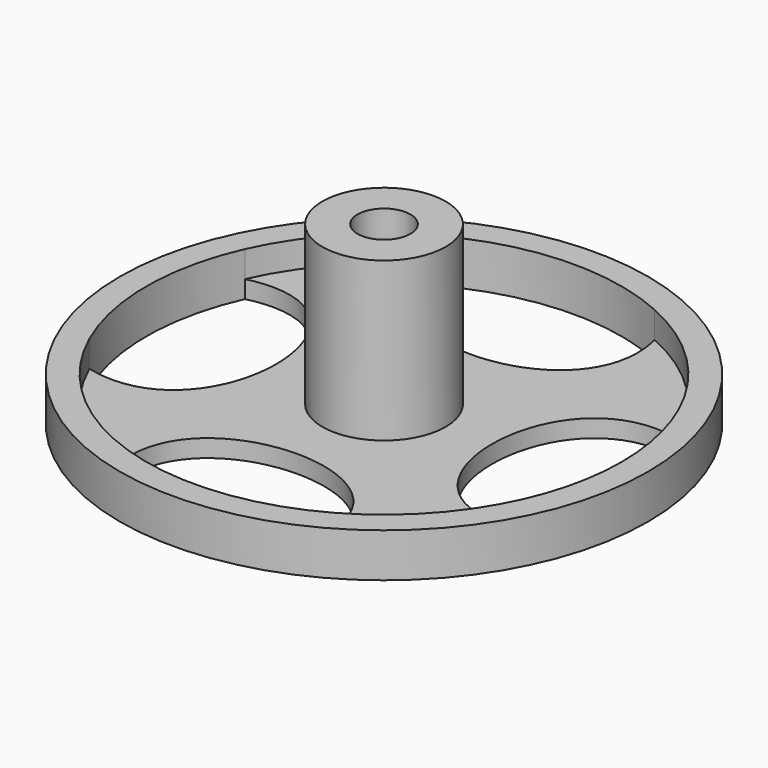
from build123d import *

# Parameters (mm, degrees)
F0_R     = 30
F1_DEPTH = 5
F0_R_2   = 7
F0_R_3   = 3
F2_DEPTH = 2
F3_DEPTH = 15


# Not quite as in the source:
# - a feature names something its author has since deleted; it is built from what else it names


with BuildPart() as f1:
    # F0 (on Top) → F1 (new body)
    with BuildSketch(Plane.XY):
        Circle(F0_R)
        with BuildLine():
            ThreePointArc((24.6394529882, 11.040713584), (26.4032690275, 5.6451204292), (27, 0))
            ThreePointArc((27, 0), (26.4032690275, -5.6451204292), (24.6394529882, -11.040713584))
            ThreePointArc((24.6394529882, -11.040713584), (19.091883092, -19.091883092), (11.040713584, -24.6394529882))
            ThreePointArc((11.040713584, -24.6394529882), (0, -27), (-11.040713584, -24.6394529882))
            ThreePointArc((-11.040713584, -24.6394529882), (-19.091883092, -19.091883092), (-24.6394529882, -11.040713584))
            ThreePointArc((-24.6394529882, -11.040713584), (-27, 0), (-24.6394529882, 11.040713584))
            ThreePointArc((-24.6394529882, 11.040713584), (-19.091883092, 19.091883092), (-11.040713584, 24.6394529882))
            ThreePointArc((-11.040713584, 24.6394529882), (0, 27), (11.040713584, 24.6394529882))
            ThreePointArc((11.040713584, 24.6394529882), (19.091883092, 19.091883092), (24.6394529882, 11.040713584))
        make_face(mode=Mode.SUBTRACT)
    extrude(amount=F1_DEPTH)


with BuildPart() as f1b:
    # F0 (on Top) → F1, piece 2 (new body)
    with BuildSketch(Plane.XY):
        Circle(F0_R_2)
        Circle(F0_R_3, mode=Mode.SUBTRACT)
    extrude(amount=F1_DEPTH)

    # F3 (add): a face of the model
    f3_faces = [f1b.faces().sort_by_distance(p)[0] for p in [
        (-6.8020101013, 0, 5),
    ]]
    extrude(f3_faces, amount=F3_DEPTH)


with BuildPart() as f2:
    # F0 (on Top) → F2 (new body)
    with BuildSketch(Plane.XY):
        with BuildLine():
            add(Edge.make_bspline(
                [(24.6394529882, 11.040713584), (8.1415599535, 15), (8.1415599535, -15), (24.6394529882, -11.040713584)],
                knots=[0, 0, 0, 0, 22.081427168, 22.081427168, 22.081427168, 22.081427168], degree=3))
            ThreePointArc((24.6394529882, 11.040713584), (19.091883092, 19.091883092), (11.040713584, 24.6394529882))
            add(Edge.make_bspline(
                [(-11.040713584, 24.6394529882), (-15, 8.1415599535), (15, 8.1415599535), (11.040713584, 24.6394529882)],
                knots=[0, 0, 0, 0, 22.081427168, 22.081427168, 22.081427168, 22.081427168], degree=3))
            ThreePointArc((-11.040713584, 24.6394529882), (-19.091883092, 19.091883092), (-24.6394529882, 11.040713584))
            add(Edge.make_bspline(
                [(-24.6394529882, -11.040713584), (-8.1415599535, -15), (-8.1415599535, 15), (-24.6394529882, 11.040713584)],
                knots=[0, 0, 0, 0, 22.081427168, 22.081427168, 22.081427168, 22.081427168], degree=3))
            ThreePointArc((-24.6394529882, -11.040713584), (-19.091883092, -19.091883092), (-11.040713584, -24.6394529882))
            add(Edge.make_bspline(
                [(-11.040713584, -24.6394529882), (-15, -8.1415599535), (15, -8.1415599535), (11.040713584, -24.6394529882)],
                knots=[0, 0, 0, 0, 22.081427168, 22.081427168, 22.081427168, 22.081427168], degree=3))
            ThreePointArc((11.040713584, -24.6394529882), (19.091883092, -19.091883092), (24.6394529882, -11.040713584))
        make_face()
        Circle(F0_R_2, mode=Mode.SUBTRACT)
    extrude(amount=F2_DEPTH)


solid = Compound([f1.part, f1b.part, f2.part])
